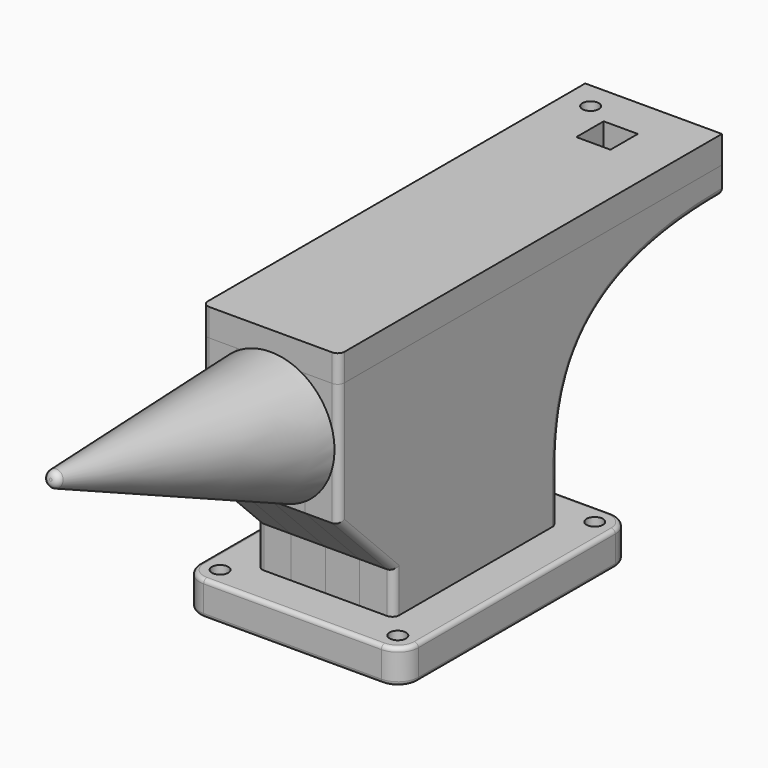
from build123d import *

# Parameters (mm, degrees)
F1_DEPTH  = 25
F4_W      = 160
F4_H      = 210
F5_DEPTH  = 25
F6_W      = 100
F6_H      = 350
F7_DEPTH  = 20
F11_R     = 6
F12_DEPTH = 25.001
F13_R     = 15
F14_R     = 3
F15_R     = 5
F15_2_R   = 5
F15_3_R   = 5
F15_4_R   = 5
F15_5_R   = 5
F15_6_R   = 5
F16_W     = 25
F16_H     = 25
F17_DEPTH = 215.001
F18_R     = 6
F19_DEPTH = 215.001


# Not quite as in the source:
# - a pattern or mirror of a feature is missing from the dataset's text; its kind, count and spacing are read off the source's solid


with BuildPart() as f1:
    # F0 (on Right) → F1 (new body)
    with BuildSketch(Plane.YZ):
        with BuildLine():
            Line((-75, 30), (-75, 0))
            Line((-75, 0), (75, 0))
            Line((75, 0), (75, 30))
            add(Edge.make_bspline(
                [(225, 150), (85, 150), (75, 85), (75, 30)],
                knots=[0, 0, 0, 0, 192.093727123, 192.093727123, 192.093727123, 192.093727123], degree=3))
            Line((225, 150), (225, 170))
            Line((225, 170), (-125, 170))
            Line((-125, 170), (-125, 80))
            Line((-125, 80), (-75, 30))
        make_face()
    extrude(amount=F1_DEPTH)


with BuildPart() as f2_1:
    # F2: copy of F1
    add(f1.part.moved(Location((25, 0, 0))))


with BuildPart() as f3_1:
    # F3: instance of F2_1
    add(f2_1.part.mirror(Plane.YZ))


with BuildPart() as f3_2:
    # F3: instance of F1
    add(f1.part.mirror(Plane.YZ))


with BuildPart() as f5:
    # F4 (on Top) → F5 (new body)
    with BuildSketch(Plane.XY):
        Rectangle(F4_W, F4_H)
    extrude(amount=-F5_DEPTH)

    # F11 (on face) → F12 (cut, through all)
    with BuildSketch(Plane.XY):
        with Locations((65, -90)):
            Circle(F11_R)
    f12 = extrude(amount=-F12_DEPTH, mode=Mode.SUBTRACT)

    # F12_copies: F12 across plane
    add(f12.mirror(Plane(origin=(0, 0, 0), x_dir=(0.8106792284, 0.5854905538, 0), z_dir=(-0.5854905538, 0.8106792284, 0))), mode=Mode.SUBTRACT)

    # F12_copies1: F12 across plane
    add(f12.mirror(Plane.ZX), mode=Mode.SUBTRACT)

    # F12_copies2: F12 across plane
    add(f12.mirror(Plane(origin=(0, 0, 0), x_dir=(0, 0, -1), z_dir=(-1, 0, 0))), mode=Mode.SUBTRACT)

    # F13
    f13_edges = [f5.edges().sort_by_distance(p)[0] for p in [
        (80, 105, -12.5),
        (80, -105, -12.5),
        (-80, 105, -12.5),
        (-80, -105, -12.5),
    ]]
    fillet(f13_edges, radius=F13_R)

    # F14
    f14_edges = [f5.edges().sort_by_distance(p)[0] for p in [
        (80, 0, 0),
        (0, -105, 0),
        (0, 105, 0),
        (-80, 0, 0),
        (80, 0, -25),
        (0, 105, -25),
        (0, -105, -25),
        (-80, 0, -25),
        (-75.606602, 100.606602, 0),
        (-75.606602, -100.606602, 0),
        (75.606602, 100.606602, 0),
        (75.606602, -100.606602, 0),
        (-75.606602, 100.606602, -25),
        (-75.606602, -100.606602, -25),
        (75.606602, 100.606602, -25),
        (75.606602, -100.606602, -25),
    ]]
    fillet(f14_edges, radius=F14_R)


with BuildPart() as f7:
    # F6 (on face) → F7 (new body)
    with BuildSketch(Plane.XY.offset(170)):
        with Locations((0, 50)):
            Rectangle(F6_W, F6_H)
    extrude(amount=F7_DEPTH)


with BuildPart() as f9:
    # F8 (on Right) → F9 (revolve)
    with BuildSketch(Plane.YZ):
        Polygon((-125, 80), (-125, 130), (-326.0946743439, 175.1213026246), (-327.1893486877, 170.2426052492), align=None)
    revolve(axis=Axis((0, -225.5473371719, 152.5606513123), (0, -0.9757394751, 0.2189348688)))

    # F10: cut F3_1, F3_2, F1, F2_1, F7
    add(f3_1.part, mode=Mode.SUBTRACT)
    add(f3_2.part, mode=Mode.SUBTRACT)
    add(f1.part, mode=Mode.SUBTRACT)
    add(f2_1.part, mode=Mode.SUBTRACT)
    add(f7.part, mode=Mode.SUBTRACT)

    # F15#6
    f15_6_edges = [f9.edges().sort_by_distance(p)[0] for p in [
        (0, -325, 180),
    ]]
    fillet(f15_6_edges, radius=F15_6_R)


with BuildPart() as f1_1:
    add(f1.part)

    # F15
    f15_edges = [f1_1.edges().sort_by_distance(p)[0] for p in [
        (12.5, 225, 150),
    ]]
    fillet(f15_edges, radius=F15_R)


with BuildPart() as f2_1_1:
    add(f2_1.part)

    # F15#2
    f15_2_edges = [f2_1_1.edges().sort_by_distance(p)[0] for p in [
        (50, 117.197501, 127.281735),
        (37.5, 225, 150),
        (50, -75, 15),
        (50, -100, 55),
        (50, -125, 125),
        (50, 75, 15),
    ]]
    fillet(f15_2_edges, radius=F15_2_R)


with BuildPart() as f3_1_1:
    add(f3_1.part)

    # F15#3
    f15_3_edges = [f3_1_1.edges().sort_by_distance(p)[0] for p in [
        (-50, 117.197501, 127.281735),
        (-37.5, 225, 150),
        (-50, -75, 15),
        (-50, -100, 55),
        (-50, -125, 125),
        (-50, 75, 15),
    ]]
    fillet(f15_3_edges, radius=F15_3_R)


with BuildPart() as f3_2_1:
    add(f3_2.part)

    # F15#4
    f15_4_edges = [f3_2_1.edges().sort_by_distance(p)[0] for p in [
        (-12.5, 225, 150),
    ]]
    fillet(f15_4_edges, radius=F15_4_R)


with BuildPart() as f7_1:
    add(f7.part)

    # F15#5
    f15_5_edges = [f7_1.edges().sort_by_distance(p)[0] for p in [
        (50, -125, 180),
        (-50, -125, 180),
    ]]
    fillet(f15_5_edges, radius=F15_5_R)


with BuildPart() as f17_tool:
    # F16 (on face) → F17 (new body, through all)
    with BuildSketch(Plane.XY.offset(190)):
        with Locations((0, 182.5)):
            Rectangle(F16_W, F16_H)
    extrude(amount=-F17_DEPTH)


with BuildPart() as f1_2:
    add(f1_1.part)

    # F17: cut by f17_tool
    add(f17_tool.part, mode=Mode.SUBTRACT)


with BuildPart() as f3_2_2:
    add(f3_2_1.part)

    # F17: cut by f17_tool
    add(f17_tool.part, mode=Mode.SUBTRACT)


with BuildPart() as f7_2:
    add(f7_1.part)

    # F17: cut by f17_tool
    add(f17_tool.part, mode=Mode.SUBTRACT)


with BuildPart() as f19_tool:
    # F18 (on face) → F19 (new body, through all)
    with BuildSketch(Plane.XY.offset(190)):
        with Locations((-30, 205)):
            Circle(F18_R)
    extrude(amount=-F19_DEPTH)


with BuildPart() as f3_1_2:
    add(f3_1_1.part)

    # F19: cut by f19_tool
    add(f19_tool.part, mode=Mode.SUBTRACT)


with BuildPart() as f3_2_3:
    add(f3_2_2.part)

    # F19: cut by f19_tool
    add(f19_tool.part, mode=Mode.SUBTRACT)


with BuildPart() as f7_3:
    add(f7_2.part)

    # F19: cut by f19_tool
    add(f19_tool.part, mode=Mode.SUBTRACT)


solid = Compound([f5.part, f9.part, f2_1_1.part, f1_2.part, f3_1_2.part, f3_2_3.part, f7_3.part])
